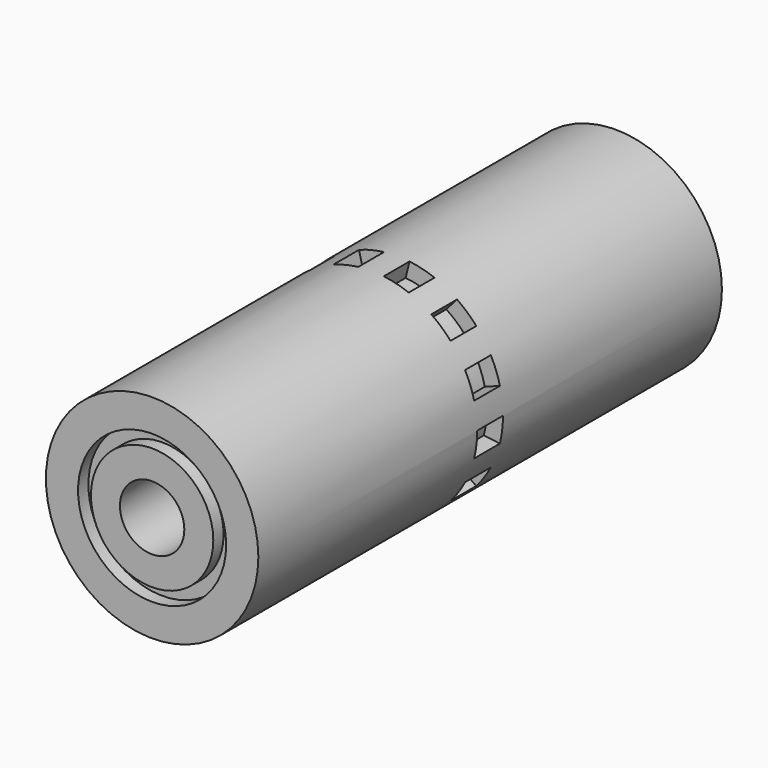
from build123d import *

# Parameters (mm, degrees)
F0_R            = 16.5
F1_DEPTH        = 90
F2_R            = 10.25
F3_DEPTH        = 25
F6_W            = 2
F6_H            = 5
F7_DEPTH        = 25
F7_COPIES_COUNT = 13
F8_R            = 14
F9_DEPTH        = 53.8
F10_R           = 8.5
F11_DEPTH       = 24.9
F4_R            = 11.5
F12_DEPTH       = 2
F13_R           = 9.5
F13_R_2         = 3.5
F5_R            = 3.5
F14_DEPTH       = 4.1
F15_R           = 5
F16_DEPTH       = 92.2


# Not quite as in the source:
# - a pattern or mirror of a feature is missing from the dataset's text; its kind, count and spacing are read off the source's solid


with BuildPart() as f1:
    # F0 (on Front) → F1 (new body)
    with BuildSketch(Plane.XZ):
        Circle(F0_R)
    extrude(amount=F1_DEPTH)

    # F2 (on face) → F3 (cut)
    with BuildSketch(Plane(origin=(0, 0, 0), x_dir=(-1, 0, 0), z_dir=(0, 1, 0))):
        Circle(F2_R)
    extrude(amount=-F3_DEPTH, mode=Mode.SUBTRACT)

    # F6 (on Top) → F7 (cut)
    with BuildSketch(Plane.XY):
        with Locations((1, -45)):
            Rectangle(F6_W, F6_H)
        with Locations((-1, -45)):
            Rectangle(F6_W, F6_H)
    f7 = extrude(amount=-F7_DEPTH, mode=Mode.SUBTRACT)

    # F7_copies: F7 ×13 about axis
    f7_copies_axis = Axis((0, 0, 0), (0, 1, 0))
    for i in range(1, F7_COPIES_COUNT):
        add(f7.rotate(f7_copies_axis, i * 360 / F7_COPIES_COUNT), mode=Mode.SUBTRACT)

    # F8 (on face) → F9 (join)
    with BuildSketch(Plane.XZ.offset(90)):
        Circle(F8_R)
    extrude(amount=-F9_DEPTH)

    # F10 (on face) → F11 (join)
    with BuildSketch(Plane.XZ.offset(90)):
        Circle(F10_R)
    extrude(amount=-F11_DEPTH)

    # F4 (on face) → F12 (cut)
    with BuildSketch(Plane.XZ.offset(90)):
        Circle(F4_R)
    extrude(amount=-F12_DEPTH, mode=Mode.SUBTRACT)

    # F13 (on face) + F5 (on face) → F14 (join)
    with BuildSketch(Plane.XZ.offset(90)):
        Circle(F13_R)
        Circle(F13_R_2, mode=Mode.SUBTRACT)
    with BuildSketch(Plane.XZ.offset(90)):
        Circle(F5_R)
    extrude(amount=-F14_DEPTH)

    # F15 (on face) → F16 (cut)
    with BuildSketch(Plane.XZ.offset(90)):
        Circle(F15_R)
    extrude(amount=-F16_DEPTH, mode=Mode.SUBTRACT)


solid = f1.part
